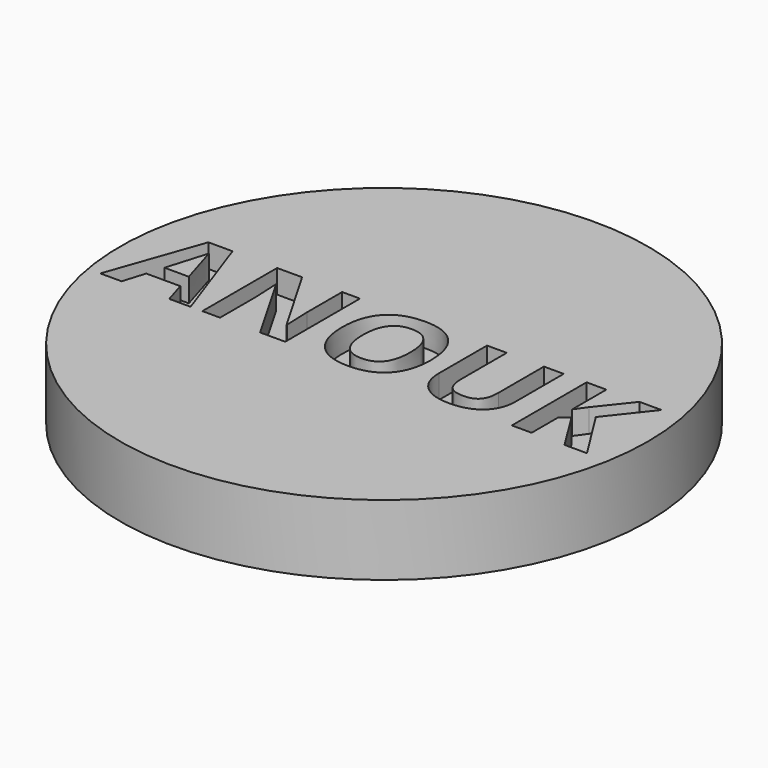
from build123d import *

# Parameters (mm, degrees)
F0_R         = 11.25
F1_DEPTH     = 3
F2_TEXT_SIZE = 5.5777387728
F3_DEPTH     = 1


# Not quite as in the source:
# - Text() gives the source's letters only with a copy of the font that has no kerning and outlines rounded to 1/6400 em; it was checked with that copy


with BuildPart() as f1:
    # F0 (on Top) → F1 (new body)
    with BuildSketch(Plane.XY):
        Circle(F0_R)
    extrude(amount=F1_DEPTH)

    # F2 (on face) → F3 (cut)
    with BuildSketch(Plane.XY.offset(3)):
        with Locations((-10.5523845408, -1.9288929861)):
            Text('ANOUK', F2_TEXT_SIZE, font='Open Sans', font_style=FontStyle.BOLD, text_align=(TextAlign.LEFT, TextAlign.BOTTOM))
    extrude(amount=-F3_DEPTH, mode=Mode.SUBTRACT)


solid = f1.part
